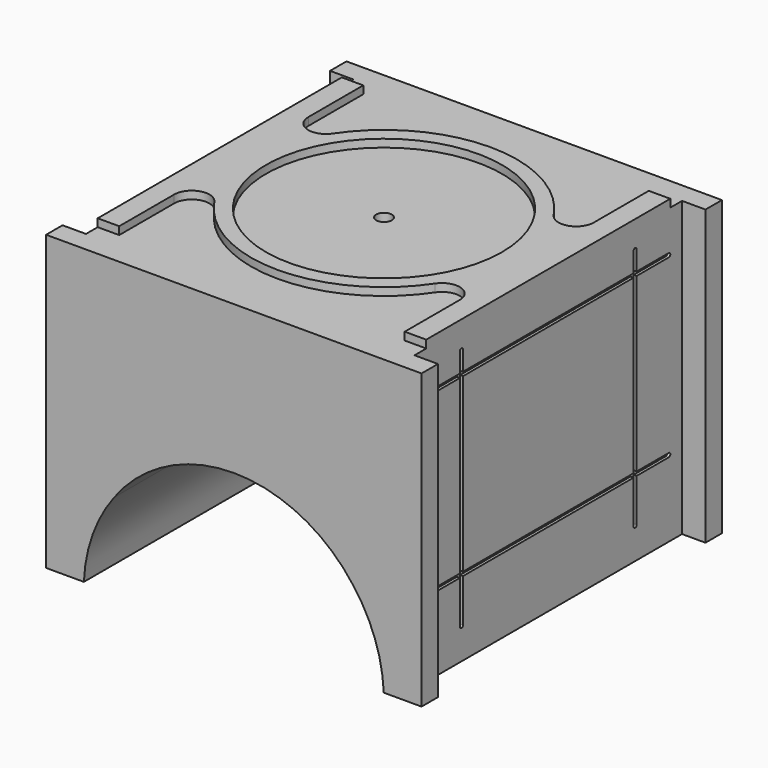
from build123d import *

# Parameters (mm, degrees)
F0_W      = 609.6
F0_H      = 609.6
F1_DEPTH  = 238.125
F3_DEPTH  = 609.601
F4_W      = 76.2
F4_H      = 542.925
F5_DEPTH  = 476.251
F6_R      = 191.690625
F7_DEPTH  = 12.7
F9_D      = 25.4
F9_DEPTH  = 34.925
F9_TIP    = 7.6309298617
F10_W     = 346.075
F10_H     = 279.4
F11_DEPTH = 4.7625


# Not quite as in the source:
# - a pattern or mirror of a feature is missing from the dataset's text; its kind, count and spacing are read off the source's solid


with BuildPart() as f1:
    # F0 (on Top) → F1 (new body, symmetric)
    with BuildSketch(Plane.XY):
        Rectangle(F0_W, F0_H)
    extrude(amount=F1_DEPTH, both=True)

    # F2 (on face) → F3 (cut, through all)
    with BuildSketch(Plane.XZ.offset(304.8)):
        with BuildLine():
            ThreePointArc((-193.9860043921, -100.965), (-230.9234761066, -170.6305134371), (-243.68125, -248.44375))
            Line((-243.68125, -248.44375), (243.68125, -248.44375))
            ThreePointArc((243.68125, -248.44375), (230.9234761066, -170.6305134371), (193.9860043921, -100.965))
            ThreePointArc((193.9860043921, -100.965), (0, -3.175), (-193.9860043921, -100.965))
        make_face()
    extrude(amount=-F3_DEPTH, mode=Mode.SUBTRACT)

    # F4 (on face) → F5 (cut, through all)
    with BuildSketch(Plane.XY.offset(238.125)):
        with Locations((304.8, 0)):
            Rectangle(F4_W, F4_H)
        with Locations((-304.8, 0)):
            Rectangle(F4_W, F4_H)
    extrude(amount=-F5_DEPTH, mode=Mode.SUBTRACT)

    # F6 (on face) → F7 (join)
    with BuildSketch(Plane.XY.offset(238.125)):
        with BuildLine():
            ThreePointArc((-231.775, -136.128125), (-211.4711543972, -108.732394395), (-179.3535020392, -120.1878999995))
            ThreePointArc((-179.3535020392, -120.1878999995), (0, -215.9), (179.3535020392, -120.1878999995))
            ThreePointArc((179.3535020392, -120.1878999995), (211.4711543972, -108.732394395), (231.775, -136.128125))
            Line((231.775, -136.128125), (231.775, -247.65))
            Line((231.775, -247.65), (266.7, -247.65))
            Line((266.7, -247.65), (266.7, 247.65))
            Line((266.7, 247.65), (231.775, 247.65))
            Line((231.775, 247.65), (231.775, 136.128125))
            ThreePointArc((231.775, 136.128125), (211.4711543972, 108.732394395), (179.3535020392, 120.1878999995))
            ThreePointArc((179.3535020392, 120.1878999995), (0, 215.9), (-179.3535020392, 120.1878999995))
            ThreePointArc((-179.3535020392, 120.1878999995), (-211.4711543972, 108.732394395), (-231.775, 136.128125))
            Line((-231.775, 136.128125), (-231.775, 247.65))
            Line((-231.775, 247.65), (-266.7, 247.65))
            Line((-266.7, 247.65), (-266.7, -247.65))
            Line((-266.7, -247.65), (-231.775, -247.65))
            Line((-231.775, -247.65), (-231.775, -136.128125))
        make_face()
        Circle(F6_R, mode=Mode.SUBTRACT)
    extrude(amount=F7_DEPTH)

    # F9
    with Locations(Plane.XY.offset(238.125)):
        with Locations((0, 0)):
            Hole(F9_D / 2, depth=F9_DEPTH)
            with Locations((0, 0, -(F9_DEPTH + F9_TIP / 2))):  # 118° drill point
                Cone(0, F9_D / 2, F9_TIP, mode=Mode.SUBTRACT)

    # F10 (on face) → F11 (cut)
    with BuildSketch(Plane.YZ.offset(266.7)):
        with BuildLine():
            Line((179.3875, -117.475), (244.475, -117.475))
            ThreePointArc((244.475, -117.475), (247.65, -114.3), (244.475, -111.125))
            Line((244.475, -111.125), (179.3875, -111.125))
            Line((179.3875, -111.125), (179.3875, 168.275))
            Line((179.3875, 168.275), (244.475, 168.275))
            ThreePointArc((244.475, 168.275), (247.65, 171.45), (244.475, 174.625))
            Line((244.475, 174.625), (179.3875, 174.625))
            Line((179.3875, 174.625), (179.3875, 206.375))
            ThreePointArc((179.3875, 206.375), (176.2125, 209.55), (173.0375, 206.375))
            Line((173.0375, 206.375), (173.0375, 174.625))
            Line((173.0375, 174.625), (-173.0375, 174.625))
            Line((-173.0375, 174.625), (-173.0375, 206.375))
            ThreePointArc((-173.0375, 206.375), (-176.2125, 209.55), (-179.3875, 206.375))
            Line((-179.3875, 206.375), (-179.3875, 174.625))
            Line((-179.3875, 174.625), (-244.475, 174.625))
            ThreePointArc((-244.475, 174.625), (-247.65, 171.45), (-244.475, 168.275))
            Line((-244.475, 168.275), (-179.3875, 168.275))
            Line((-179.3875, 168.275), (-179.3875, -111.125))
            Line((-179.3875, -111.125), (-244.475, -111.125))
            ThreePointArc((-244.475, -111.125), (-247.65, -114.3), (-244.475, -117.475))
            Line((-244.475, -117.475), (-179.3875, -117.475))
            Line((-179.3875, -117.475), (-179.3875, -187.325))
            ThreePointArc((-179.3875, -187.325), (-176.2125, -190.5), (-173.0375, -187.325))
            Line((-173.0375, -187.325), (-173.0375, -117.475))
            Line((-173.0375, -117.475), (173.0375, -117.475))
            Line((173.0375, -117.475), (173.0375, -187.325))
            ThreePointArc((173.0375, -187.325), (176.2125, -190.5), (179.3875, -187.325))
            Line((179.3875, -187.325), (179.3875, -117.475))
        make_face()
        with Locations((0, 28.575)):
            Rectangle(F10_W, F10_H, mode=Mode.SUBTRACT)
    f11 = extrude(amount=-F11_DEPTH, mode=Mode.SUBTRACT)

    # F11_copies: F11 across plane
    add(f11.mirror(Plane(origin=(0, 0, 0), x_dir=(0, 0, -1), z_dir=(-1, 0, 0))), mode=Mode.SUBTRACT)


solid = f1.part
